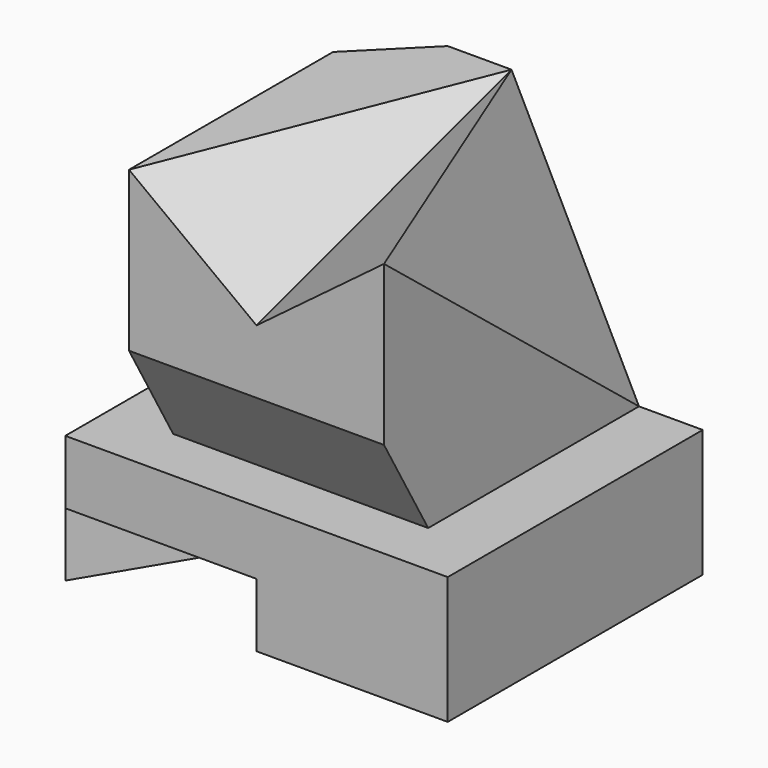
from build123d import *

# Parameters (mm, degrees)
F0_W      = 60
F0_H      = 50
F1_DEPTH  = 20
F4_DEPTH  = 10
F5_W      = 40
F5_H      = 50
F6_DEPTH  = 40
F7_SIZE   = 10
F9_DEPTH  = 40
F16_DEPTH = 16.8440384213


with BuildPart() as f1:
    # F0 (on Top) → F1 (new body)
    with BuildSketch(Plane.XY):
        with Locations((30, 25)):
            Rectangle(F0_W, F0_H)
    extrude(amount=F1_DEPTH)

    # F3 (on face) → F4 (cut, through all)
    with BuildSketch(Plane(origin=(0, 0, 0), x_dir=(1, 0, 0), z_dir=(0, 0, -1))):
        Polygon((30, 0), (0, 0), (30, -50), (60, -50), align=None)
    extrude(amount=-F4_DEPTH, mode=Mode.SUBTRACT)

    # F5 (on face) → F6 (join)
    with BuildSketch(Plane.XY.offset(20)):
        with Locations((30, 25)):
            Rectangle(F5_W, F5_H)
    extrude(amount=F6_DEPTH)

    # F7
    f7_edges = [f1.edges().sort_by_distance(p)[0] for p in [
        (10, 50, 40),
    ]]
    chamfer(f7_edges, length=F7_SIZE)

    # F8 (on face) → F9 (cut, through all)
    with BuildSketch(Plane.YZ.offset(50)):
        Polygon((0, 35), (0, 20), (8.6602540378, 20), align=None)
    extrude(amount=-F9_DEPTH, mode=Mode.SUBTRACT)

    # F13: sweep along a path in F11
    with BuildLine(Plane(origin=(30, 0, 0), x_dir=(0, -1, 0), z_dir=(-1, 0, 0))) as f13_path:
        Line((0, 45), (-50, 60))
    # F12 (on face) → F13 (sweep, cut)
    with BuildSketch(Plane.XZ):
        Polygon((50, 60), (10, 60), (30, 45), align=None)
    sweep(path=f13_path.line, mode=Mode.SUBTRACT)

    # F15 (on face) → F16 (cut, through all)
    with BuildSketch(Plane(origin=(56.7375886525, 22.695035461, 28.3687943262), x_dir=(0.3012974309, -0.9415544714, 0.1506487154), z_dir=(-0.8421519211, -0.3368607684, -0.4210759605))):
        Polygon((-28.9998777205, -4.472135955), (24.103794469, 31.304951685), (-28.9998777205, 40.249223595), align=None)
    extrude(amount=-F16_DEPTH, mode=Mode.SUBTRACT)


solid = f1.part
